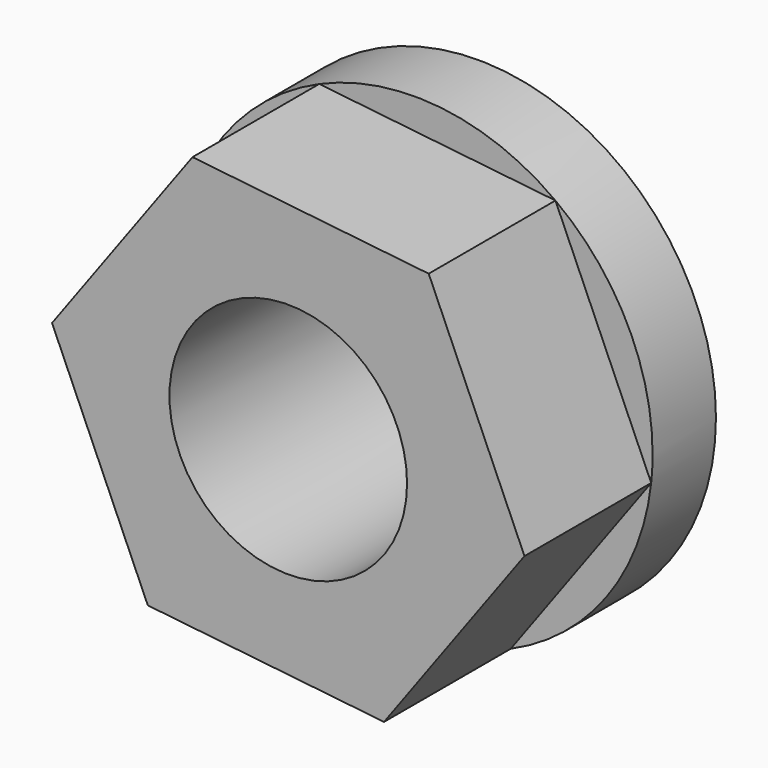
from build123d import *

# Parameters (mm, degrees)
F0_R     = 9.525
F0_R_2   = 4.7625
F1_DEPTH = 3.175
F2_R     = 4.7625
F3_DEPTH = 6.35


# Not quite as in the source:
# - a feature names something its author has since deleted; it is built from what else it names


with BuildPart() as f1:
    # F0 (on Front) → F1 (new body)
    with BuildSketch(Plane.XZ):
        with Locations((-49.2760017514, 2.0293546841)):
            Circle(F0_R)
        with Locations((-49.2760017514, 2.0293546841)):
            Circle(F0_R_2, mode=Mode.SUBTRACT)
    extrude(amount=F1_DEPTH)

    # F2 (on face) → F3 (join)
    with BuildSketch(Plane.XZ.offset(3.175)):
        Polygon((-39.8072749816, 0.9955082934), (-43.6463011287, 9.7125894129), (-53.1150278984, 10.7464358035), (-58.7447285212, 3.0632010747), (-54.9057023742, -5.6538800448), (-45.4369756044, -6.6877264354), align=None)
        with Locations((-49.2760017514, 2.0293546841)):
            Circle(F2_R, mode=Mode.SUBTRACT)
    extrude(amount=F3_DEPTH)


solid = f1.part
